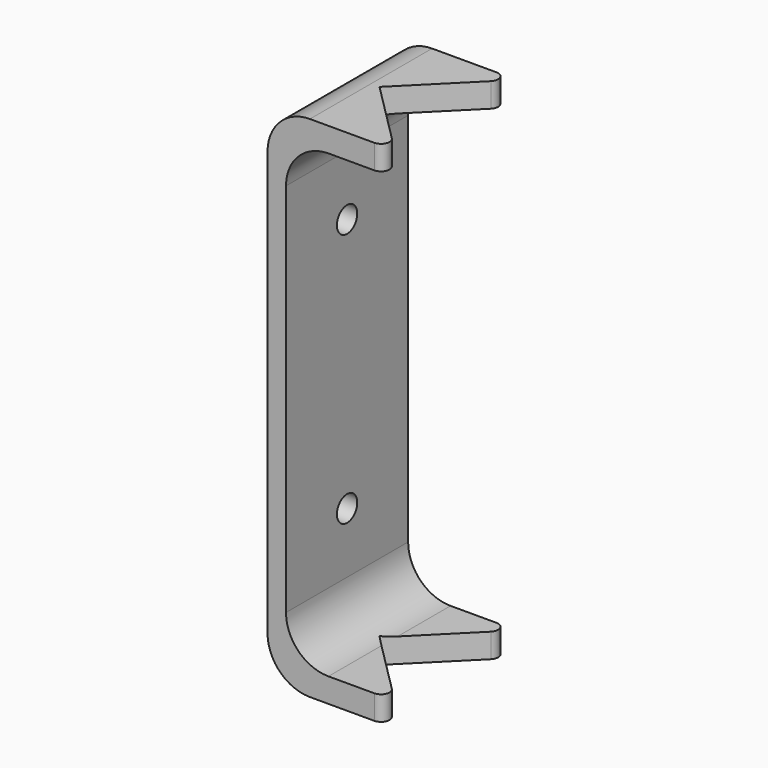
from build123d import *

# Parameters (mm, degrees)
F0_W         = 18
F0_H         = 60
F0_R         = 1.5
F1_DEPTH     = 15
F3_DEPTH     = 80
F4_W         = 12.820621879
F4_H         = 54.2796626687
F5_DEPTH     = 25
F6_R         = 1
F7_T4_DEPTH  = 18
F7_T10_DEPTH = 18
F7_T16_DEPTH = 18
F7_T22_DEPTH = 18
F7_T28_DEPTH = 18
F7_T34_DEPTH = 18
F7_T37_DEPTH = 43


# Not quite as in the source:
# - a fillet or chamfer that OpenCascade refuses, or shapes differently, is made with other operations: its cross-section is extruded or revolved along the edge and cut away or added


with BuildPart() as f1:
    # F0 (on Right) → F1 (new body)
    with BuildSketch(Plane.YZ):
        Rectangle(F0_W, F0_H)
        with Locations((0, -15)):
            Circle(F0_R, mode=Mode.SUBTRACT)
        with Locations((0, 15)):
            Circle(F0_R, mode=Mode.SUBTRACT)
    extrude(amount=F1_DEPTH)

    # F2 (on face) → F3 (cut)
    with BuildSketch(Plane.XY.offset(30)):
        Polygon((15, -9), (15, 9), (6, 0), align=None)
    extrude(amount=-F3_DEPTH, mode=Mode.SUBTRACT)

    # F4 (on face) → F5 (cut)
    with BuildSketch(Plane.XZ.offset(9)):
        with Locations((8.5896890605, 0)):
            Rectangle(F4_W, F4_H)
    extrude(amount=-F5_DEPTH, mode=Mode.SUBTRACT)

    # F6
    f6_edges = [f1.edges().sort_by_distance(p)[0] for p in [
        (15, -9, 28.569916),
        (15, 9, 28.569916),
        (15, -9, -28.569916),
        (15, 9, -28.569916),
    ]]
    fillet(f6_edges, radius=F6_R)

    # F7: fillet of radius 5 on 4 edges, made by hand


with BuildPart() as f7_tool2:
    # F7_s3 → F7_t4 (new body)
    with BuildSketch(Plane.XZ.offset(9)):
        with BuildLine():
            ThreePointArc((7.179378121, 27.1398313344), (3.6438442151, 25.6753652403), (2.179378121, 22.1398313344))
            Line((2.179378121, 22.1398313344), (2.179378121, 27.1398313344))
            Line((2.179378121, 27.1398313344), (7.179378121, 27.1398313344))
        make_face()
    extrude(amount=-F7_T4_DEPTH)

    split(bisect_by=Plane(origin=(3, 3, 0), x_dir=(0, 0, 1), z_dir=(-0.7071067812, -0.7071067812, 0)), keep=Keep.TOP)

    split(bisect_by=Plane(origin=(3, -3, 0), x_dir=(0, 0, 1), z_dir=(0.7071067812, -0.7071067812, 0)), keep=Keep.TOP)


with BuildPart() as f1_1:
    add(f1.part)

    # F7_t1: union F7_tool2
    add(f7_tool2.part)


with BuildPart() as f7_tool8:
    # F7_s9 → F7_t10 (new body)
    with BuildSketch(Plane.XZ.offset(9)):
        with BuildLine():
            ThreePointArc((7.179378121, 27.1398313344), (3.6438442151, 25.6753652403), (2.179378121, 22.1398313344))
            Line((2.179378121, 22.1398313344), (2.179378121, 27.1398313344))
            Line((2.179378121, 27.1398313344), (7.179378121, 27.1398313344))
        make_face()
    extrude(amount=-F7_T10_DEPTH)

    split(bisect_by=Plane(origin=(3, 3, 0), x_dir=(0, 0, 1), z_dir=(-0.7071067812, -0.7071067812, 0)), keep=Keep.TOP)

    split(bisect_by=Plane(origin=(3, -3, 0), x_dir=(0, 0, 1), z_dir=(-0.7071067812, 0.7071067812, 0)), keep=Keep.TOP)


with BuildPart() as f1_2:
    add(f1_1.part)

    # F7_t7: union F7_tool8
    add(f7_tool8.part)


with BuildPart() as f7_tool14:
    # F7_s15 → F7_t16 (new body)
    with BuildSketch(Plane.XZ.offset(9)):
        with BuildLine():
            ThreePointArc((7.179378121, 27.1398313344), (3.6438442151, 25.6753652403), (2.179378121, 22.1398313344))
            Line((2.179378121, 22.1398313344), (2.179378121, 27.1398313344))
            Line((2.179378121, 27.1398313344), (7.179378121, 27.1398313344))
        make_face()
    extrude(amount=-F7_T16_DEPTH)

    split(bisect_by=Plane(origin=(3, 3, 0), x_dir=(0, 0, 1), z_dir=(0.7071067812, 0.7071067812, 0)), keep=Keep.TOP)

    split(bisect_by=Plane(origin=(3, -3, 0), x_dir=(0, 0, 1), z_dir=(-0.7071067812, 0.7071067812, 0)), keep=Keep.TOP)


with BuildPart() as f1_3:
    add(f1_2.part)

    # F7_t13: union F7_tool14
    add(f7_tool14.part)


with BuildPart() as f7_tool20:
    # F7_s21 → F7_t22 (new body)
    with BuildSketch(Plane.XZ.offset(9)):
        with BuildLine():
            ThreePointArc((2.179378121, -22.1398313344), (3.6438442151, -25.6753652403), (7.179378121, -27.1398313344))
            Line((7.179378121, -27.1398313344), (2.179378121, -27.1398313344))
            Line((2.179378121, -27.1398313344), (2.179378121, -22.1398313344))
        make_face()
    extrude(amount=-F7_T22_DEPTH)

    split(bisect_by=Plane(origin=(3, 3, 0), x_dir=(0, 0, 1), z_dir=(-0.7071067812, -0.7071067812, 0)), keep=Keep.TOP)

    split(bisect_by=Plane(origin=(3, -3, 0), x_dir=(0, 0, 1), z_dir=(0.7071067812, -0.7071067812, 0)), keep=Keep.TOP)


with BuildPart() as f1_4:
    add(f1_3.part)

    # F7_t19: union F7_tool20
    add(f7_tool20.part)


with BuildPart() as f7_tool26:
    # F7_s27 → F7_t28 (new body)
    with BuildSketch(Plane.XZ.offset(9)):
        with BuildLine():
            ThreePointArc((2.179378121, -22.1398313344), (3.6438442151, -25.6753652403), (7.179378121, -27.1398313344))
            Line((7.179378121, -27.1398313344), (2.179378121, -27.1398313344))
            Line((2.179378121, -27.1398313344), (2.179378121, -22.1398313344))
        make_face()
    extrude(amount=-F7_T28_DEPTH)

    split(bisect_by=Plane(origin=(3, 3, 0), x_dir=(0, 0, 1), z_dir=(-0.7071067812, -0.7071067812, 0)), keep=Keep.TOP)

    split(bisect_by=Plane(origin=(3, -3, 0), x_dir=(0, 0, 1), z_dir=(-0.7071067812, 0.7071067812, 0)), keep=Keep.TOP)


with BuildPart() as f1_5:
    add(f1_4.part)

    # F7_t25: union F7_tool26
    add(f7_tool26.part)


with BuildPart() as f7_tool32:
    # F7_s33 → F7_t34 (new body)
    with BuildSketch(Plane.XZ.offset(9)):
        with BuildLine():
            ThreePointArc((2.179378121, -22.1398313344), (3.6438442151, -25.6753652403), (7.179378121, -27.1398313344))
            Line((7.179378121, -27.1398313344), (2.179378121, -27.1398313344))
            Line((2.179378121, -27.1398313344), (2.179378121, -22.1398313344))
        make_face()
    extrude(amount=-F7_T34_DEPTH)

    split(bisect_by=Plane(origin=(3, 3, 0), x_dir=(0, 0, 1), z_dir=(0.7071067812, 0.7071067812, 0)), keep=Keep.TOP)

    split(bisect_by=Plane(origin=(3, -3, 0), x_dir=(0, 0, 1), z_dir=(-0.7071067812, 0.7071067812, 0)), keep=Keep.TOP)


with BuildPart() as f1_6:
    add(f1_5.part)

    # F7_t31: union F7_tool32
    add(f7_tool32.part)

    # F7_s38 → F7_t37 (cut)
    with BuildSketch(Plane.XZ.offset(-21.5)):
        with BuildLine():
            ThreePointArc((0, 25), (1.4644660941, 28.5355339059), (5, 30))
            Line((5, 30), (0, 30))
            Line((0, 30), (0, 25))
        make_face()
        with BuildLine():
            ThreePointArc((5, -30), (1.4644660941, -28.5355339059), (0, -25))
            Line((0, -25), (0, -30))
            Line((0, -30), (5, -30))
        make_face()
    extrude(amount=F7_T37_DEPTH, mode=Mode.SUBTRACT)


solid = f1_6.part
